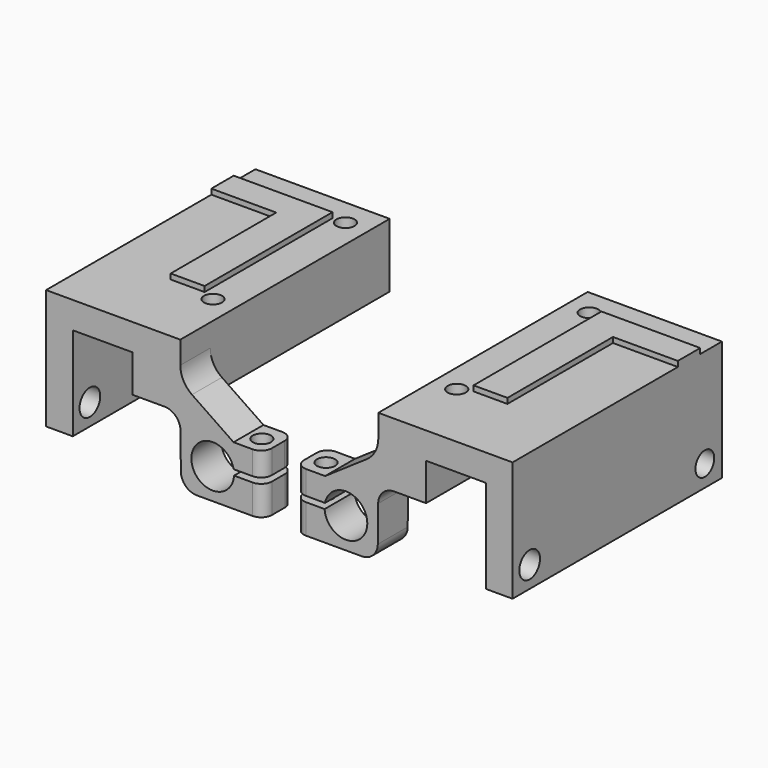
from build123d import *

# Parameters (mm, degrees)
F1_DEPTH      = 7
F2_DEPTH      = 42
F3_R          = 1.7
F3_R_2        = 11
F4_DEPTH      = 12.001
F5_R          = 4
F6_DEPTH      = 10
F7_DEPTH      = 12.001
F8_R          = 1.4
F9_DEPTH      = 10.9920075553
F8_R_2        = 1.7
F10_DEPTH     = 4.4348209087
F11_R         = 5
F12_R         = 3
F13_R         = 3
F14_R         = 2
F15_R         = 2.2
F15_R_2       = 2.4255023423
F16_DEPTH     = 6
F17_TEXT_SIZE = 41.9437823343
F18_DEPTH     = 1


# Not quite as in the source:
# - a feature names something its author has since deleted; it is built from what else it names
# - Text() gives the source's letters only with a copy of the font that has no kerning and outlines rounded to 1/6400 em; it was checked with that copy


with BuildPart() as f1:
    # F0 (on Front) → F1 (new body)
    with BuildSketch(Plane.XZ):
        Polygon((-18.6721007523, 29.8099789735), (-18.6721007523, 7.3259699669), (-13.6721007523, 7.3259699669), (-13.6721007523, 24.8099789735), (-2.4721007523, 24.8099789735), (-2.4721007523, 17.8099789735), (6.4637966118, 17.8099789735), (6.4637966118, 22.9406704692), (6.4637966118, 29.8099789735), align=None)
        Polygon((16.4301751077, 16.1394868046), (6.4637966118, 22.9406704692), (6.4637966118, 17.8099789735), (6.5940201178, 5.1484792493), (22.0186601057, 5.1484792493), (22.0186601057, 10.6682249423), (14.6860510706, 10.6682249423), (14.6860510706, 11.7046658959), (21.9896428882, 11.7046658959), (21.9896428882, 16.1394868046), align=None)
    extrude(amount=F1_DEPTH)

    # F0 (on Front) → F2 (join)
    with BuildSketch(Plane.XZ):
        Polygon((-18.6721007523, 29.8099789735), (-18.6721007523, 7.3259699669), (-13.6721007523, 7.3259699669), (-13.6721007523, 24.8099789735), (-2.4721007523, 24.8099789735), (-2.4721007523, 17.8099789735), (6.4637966118, 17.8099789735), (6.4637966118, 22.9406704692), (6.4637966118, 29.8099789735), align=None)
    extrude(amount=-F2_DEPTH)

    # F3 (on face) → F4 (cut, through all)
    with BuildSketch(Plane(origin=(0, 0, 17.8099789735), x_dir=(1, 0, 0), z_dir=(0, 0, -1))):
        with Locations((2.1850741468, -6)):
            Circle(F3_R)
        with Locations((2.1850741468, -37)):
            Circle(F3_R)
        with Locations((17.6850741468, -21.5)):
            Circle(F3_R_2)
    extrude(amount=-F4_DEPTH, mode=Mode.SUBTRACT)

    # F5 (on face) → F6 (cut)
    with BuildSketch(Plane.XZ.offset(7)):
        with Locations((12.5278992477, 10.8989789735)):
            Circle(F5_R)
    extrude(amount=-F6_DEPTH, mode=Mode.SUBTRACT)

    # F3 (on face) → F7 (cut, through all)
    with BuildSketch(Plane(origin=(0, 0, 17.8099789735), x_dir=(1, 0, 0), z_dir=(0, 0, -1))):
        with Locations((2.1850741468, -6)):
            Circle(F3_R)
        with Locations((2.1850741468, -37)):
            Circle(F3_R)
        with Locations((17.6850741468, -21.5)):
            Circle(F3_R_2)
    extrude(amount=-F7_DEPTH, mode=Mode.SUBTRACT)

    # F8 (on face) → F9 (cut, through all)
    with BuildSketch(Plane.XY.offset(16.1394868046)):
        with Locations((18.9896428882, -3.5767070949)):
            Circle(F8_R)
    extrude(amount=-F9_DEPTH, mode=Mode.SUBTRACT)

    # F8 (on face) → F10 (cut, through all)
    with BuildSketch(Plane.XY.offset(16.1394868046)):
        with Locations((18.9896428882, -3.5767070949)):
            Circle(F8_R_2)
        with Locations((18.9896428882, -3.5767070949)):
            Circle(F8_R, mode=Mode.SUBTRACT)
    extrude(amount=-F10_DEPTH, mode=Mode.SUBTRACT)

    # F11
    f11_edges = [f1.edges().sort_by_distance(p)[0] for p in [
        (6.463797, -3.5, 22.94067),
    ]]
    fillet(f11_edges, radius=F11_R)

    # F12
    f12_edges = [f1.edges().sort_by_distance(p)[0] for p in [
        (6.463797, -3.5, 17.809979),
    ]]
    fillet(f12_edges, radius=F12_R)

    # F13
    f13_edges = [f1.edges().sort_by_distance(p)[0] for p in [
        (6.59402, -3.5, 5.148479),
    ]]
    fillet(f13_edges, radius=F13_R)

    # F14
    f14_edges = [f1.edges().sort_by_distance(p)[0] for p in [
        (21.989643, -7, 13.922076),
        (22.01866, -7, 7.908352),
        (21.989643, 0, 13.922076),
        (22.01866, 0, 7.908352),
    ]]
    fillet(f14_edges, radius=F14_R)

    # F15 (on face) → F16 (cut)
    with BuildSketch(Plane(origin=(-18.6721007523, 0, 0), x_dir=(0, -1, 0), z_dir=(-1, 0, 0))):
        with Locations((-38, 11.3259699669)):
            Circle(F15_R)
        with Locations((3, 11.3259699669)):
            Circle(F15_R_2)
    extrude(amount=-F16_DEPTH, mode=Mode.SUBTRACT)

    # F17 (on face) → F18 (join)
    with BuildSketch(Plane.XY.offset(29.8099789735)):
        with Locations(Location((3.5908724648, 36.9253193088), (0, 0, 180))):
            Text('L', F17_TEXT_SIZE, font='Open Sans', font_style=FontStyle.BOLD, text_align=(TextAlign.LEFT, TextAlign.BOTTOM))
    extrude(amount=F18_DEPTH)


with BuildPart() as f19_1:
    # F19: instance of F1
    add(f1.part.mirror(Plane.YZ))


with BuildPart() as f19_1_1:
    # F20: moved
    add(f19_1.part.moved(Location((50, 0, 0))))


solid = Compound([f1.part, f19_1_1.part])
